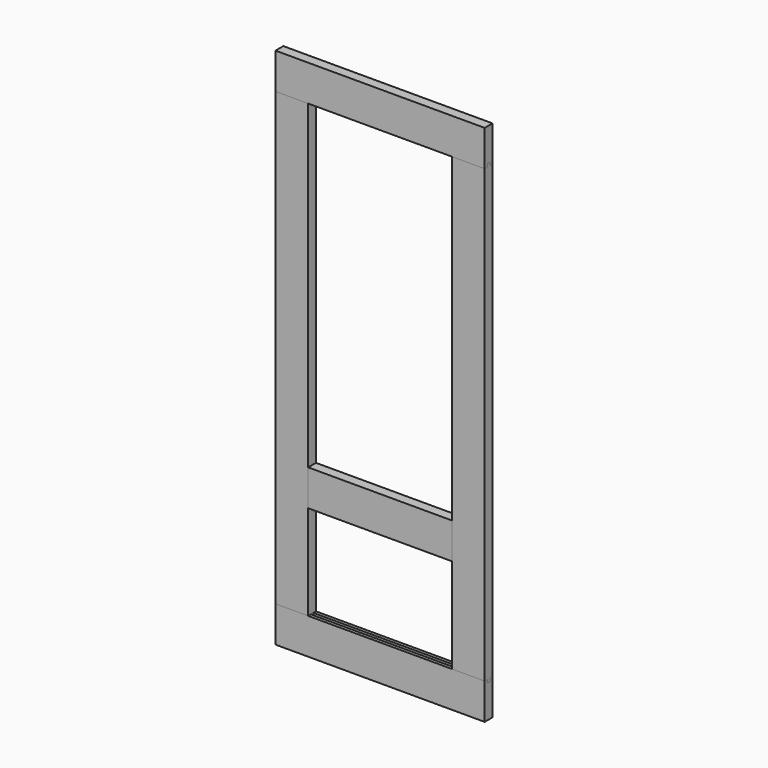
from build123d import *

# Parameters (mm, degrees)
F1_DEPTH  = 812.8
F5_DEPTH  = 127
F12_W     = 38.1
F12_H     = 139.7
F13_DEPTH = 279.4


# Not quite as in the source:
# - a feature of the source that left no trace in its solid (it failed there, or was rolled back) is left out


with BuildPart() as f1:
    # F0 (on Right) → F1 (new body)
    with BuildSketch(Plane.YZ):
        Polygon((0, 139.7), (0, 0), (38.1, 0), (38.1, 139.7), (25.4, 139.7), (25.4, 127), (12.7, 127), (12.7, 139.7), align=None)
    extrude(amount=F1_DEPTH)


with BuildPart() as f3_1:
    # F3: instance of F1
    add(f1.part.mirror(Plane.XY.offset(1016)))


with BuildPart() as f5:
    # F4 (on Right) → F5 (new body)
    with BuildSketch(Plane.YZ):
        Polygon((0, 1892.3), (0, 139.7), (12.7, 139.7), (12.7, 127), (25.4, 127), (25.4, 139.51589757), (38.1, 139.51589757), (38.1, 1892.3), (25.4, 1892.3), (25.4, 1905), (12.7, 1905), (12.7, 1892.3), align=None)
    extrude(amount=F5_DEPTH)


with BuildPart() as f7_1:
    # F7: instance of F5
    add(f5.part.mirror(Plane.YZ.offset(406.4)))


with BuildPart() as f13:
    # F12 (on offset) → F13 (new body, symmetric)
    with BuildSketch(Plane.YZ.offset(406.4)):
        with Locations((19.05, 577.85)):
            Rectangle(F12_W, F12_H)
    extrude(amount=F13_DEPTH, both=True)


solid = Compound([f1.part, f3_1.part, f5.part, f7_1.part, f13.part])
